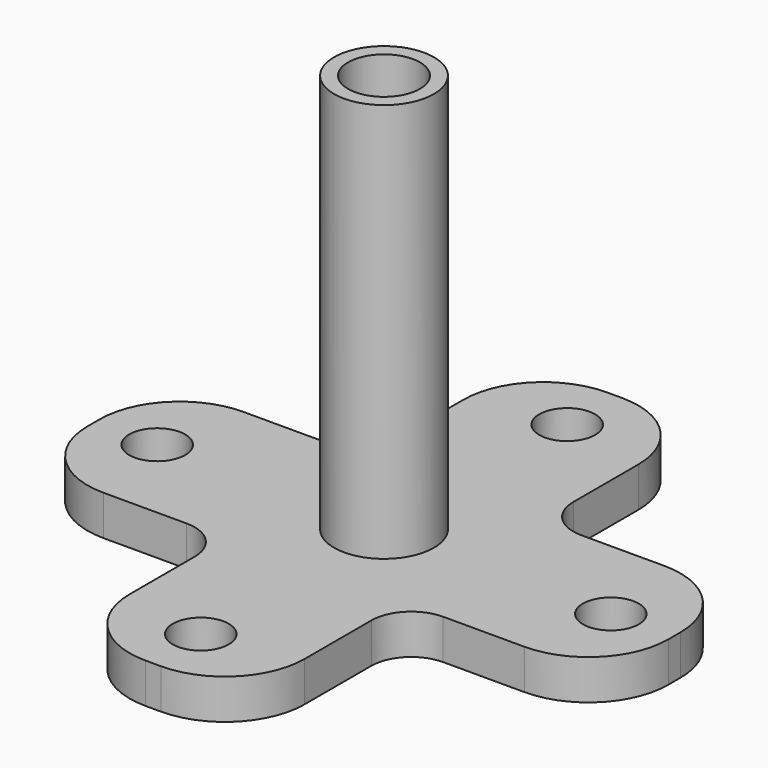
from build123d import *

# Parameters (mm, degrees)
F0_R     = 4.445
F1_DEPTH = 6.35
F2_R     = 7.9375
F2_R_2   = 5.715
F3_DEPTH = 63.5


with BuildPart() as f1:
    # F0 (on Top) → F1 (new body)
    with BuildSketch(Plane.XY):
        with BuildLine():
            Line((33.3375, 14.071082), (20.108373, 14.071082))
            ThreePointArc((20.108373, 14.071082), (15.618245, 15.930954), (13.758373, 20.421082))
            Line((13.758373, 20.421082), (13.758373, 33.3375))
            ThreePointArc((13.758373, 33.3375), (10.038629, 42.317756), (1.058373, 46.0375))
            Line((1.058373, 46.0375), (-1.371082, 46.0375))
            ThreePointArc((-1.371082, 46.0375), (-10.351338, 42.317756), (-14.071082, 33.3375))
            Line((-14.071082, 33.3375), (-14.071082, 20.108373))
            ThreePointArc((-14.071082, 20.108373), (-15.930954, 15.618245), (-20.421082, 13.758373))
            Line((-20.421082, 13.758373), (-33.3375, 13.758373))
            ThreePointArc((-33.3375, 13.758373), (-42.317756, 10.038629), (-46.0375, 1.058373))
            Line((-46.0375, 1.058373), (-46.0375, -1.371082))
            ThreePointArc((-46.0375, -1.371082), (-42.317756, -10.351338), (-33.3375, -14.071082))
            Line((-33.3375, -14.071082), (-20.108373, -14.071082))
            ThreePointArc((-20.108373, -14.071082), (-15.618245, -15.930954), (-13.758373, -20.421082))
            Line((-13.758373, -20.421082), (-13.758373, -33.3375))
            ThreePointArc((-13.758373, -33.3375), (-10.038629, -42.317756), (-1.058373, -46.0375))
            Line((-1.058373, -46.0375), (1.371082, -46.0375))
            ThreePointArc((1.371082, -46.0375), (10.351338, -42.317756), (14.071082, -33.3375))
            Line((14.071082, -33.3375), (14.071082, -20.108373))
            ThreePointArc((14.071082, -20.108373), (15.930954, -15.618245), (20.421082, -13.758373))
            Line((20.421082, -13.758373), (33.3375, -13.758373))
            ThreePointArc((33.3375, -13.758373), (42.317756, -10.038629), (46.0375, -1.058373))
            Line((46.0375, -1.058373), (46.0375, 1.371082))
            ThreePointArc((46.0375, 1.371082), (42.317756, 10.351338), (33.3375, 14.071082))
        make_face()
        with Locations((-0.170675, -36.194598)):
            Circle(F0_R, mode=Mode.SUBTRACT)
        with Locations((36.194598, -0.170675)):
            Circle(F0_R, mode=Mode.SUBTRACT)
        with Locations((-36.194598, 0.170675)):
            Circle(F0_R, mode=Mode.SUBTRACT)
        with BuildLine():
            ThreePointArc((0, 7.9375), (5.61266, 5.61266), (7.9375, 0))
            ThreePointArc((7.9375, 0), (5.61266, -5.61266), (0, -7.9375))
            ThreePointArc((0, -7.9375), (-7.9375, 0), (0, 7.9375))
        make_face(mode=Mode.SUBTRACT)
        with Locations((0.170675, 36.194598)):
            Circle(F0_R, mode=Mode.SUBTRACT)
        with BuildLine():
            ThreePointArc((0, -7.9375), (5.61266, -5.61266), (7.9375, 0))
            ThreePointArc((7.9375, 0), (5.61266, 5.61266), (0, 7.9375))
            Line((0, 7.9375), (0, 5.715))
            ThreePointArc((0, 5.715), (4.041115, 4.041115), (5.715, 0))
            ThreePointArc((5.715, 0), (4.041115, -4.041115), (0, -5.715))
            Line((0, -5.715), (0, -7.9375))
        make_face()
        with BuildLine():
            Line((0, 5.715), (0, 7.9375))
            ThreePointArc((0, 7.9375), (-7.9375, 0), (0, -7.9375))
            Line((0, -7.9375), (0, -5.715))
            ThreePointArc((0, -5.715), (-5.715, 0), (0, 5.715))
        make_face()
    extrude(amount=F1_DEPTH)

    # F2 (on face) → F3 (join)
    with BuildSketch(Plane.XY.offset(6.35)):
        Circle(F2_R)
        Circle(F2_R_2, mode=Mode.SUBTRACT)
    extrude(amount=F3_DEPTH)


solid = f1.part
